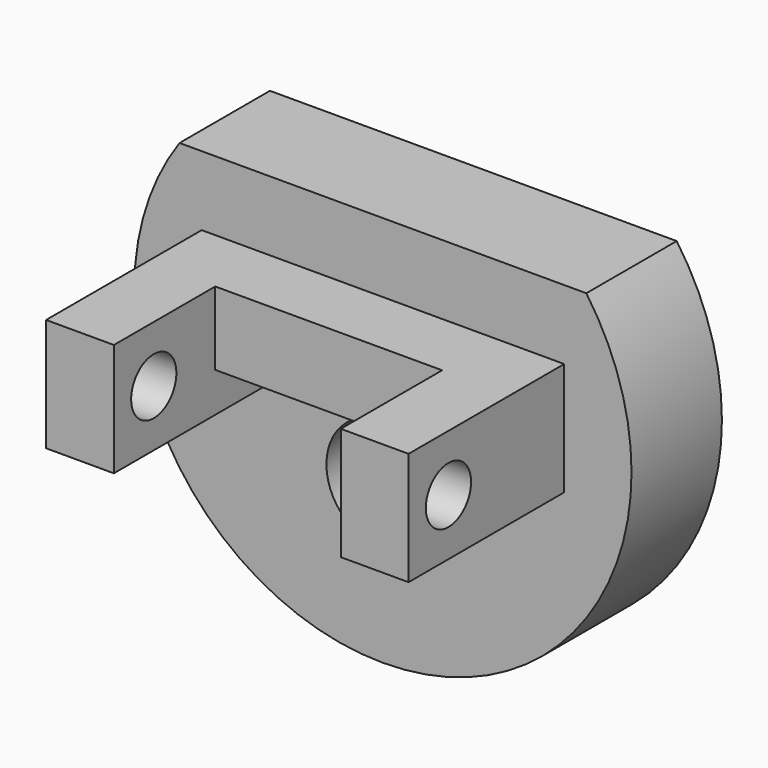
from build123d import *

# Parameters (mm, degrees)
F1_DEPTH = 6.35
F3_D     = 6.35
F2_W     = 3.81
F2_H     = 6.35
F4_DEPTH = 10.9299502
F6_D     = 3.175
F7_W     = 12.7500126
F7_H     = 4.1250048568
F8_DEPTH = 3.81


# Not quite as in the source:
# - a feature names something its author has since deleted; it is built from what else it names


with BuildPart() as f1:
    # F0 (on Front) → F1 (new body)
    with BuildSketch(Plane.XZ):
        with BuildLine():
            Line((11.43, 8.0321852568), (-11.43, 8.0321852568))
            ThreePointArc((-11.43, 8.0321852568), (0, -13.97), (11.43, 8.0321852568))
        make_face()
    extrude(amount=F1_DEPTH)

    # F3 (through all)
    with Locations(Plane.XZ.offset(6.35)):
        with Locations((0, -5.1758147432)):
            Hole(F3_D / 2)

    # F2 (on face) → F4 (join)
    with BuildSketch(Plane.XZ.offset(6.35)):
        with Locations((-8.2800063, 0.9500048568)):
            Rectangle(F2_W, F2_H)
        with Locations((8.2800063, 0.9500048568)):
            Rectangle(F2_W, F2_H)
    extrude(amount=F4_DEPTH)

    # F6 (through all)
    with Locations(Plane(origin=(-10.1850063, 0, 0), x_dir=(0, -1, 0), z_dir=(-1, 0, 0))):
        with Locations((14.478, 0.9500048568)):
            Hole(F6_D / 2)

    # F7 (on face) → F8 (join)
    with BuildSketch(Plane.XZ.offset(6.35)):
        with Locations((0, 2.0625024284)):
            Rectangle(F7_W, F7_H)
    extrude(amount=F8_DEPTH)


solid = f1.part
